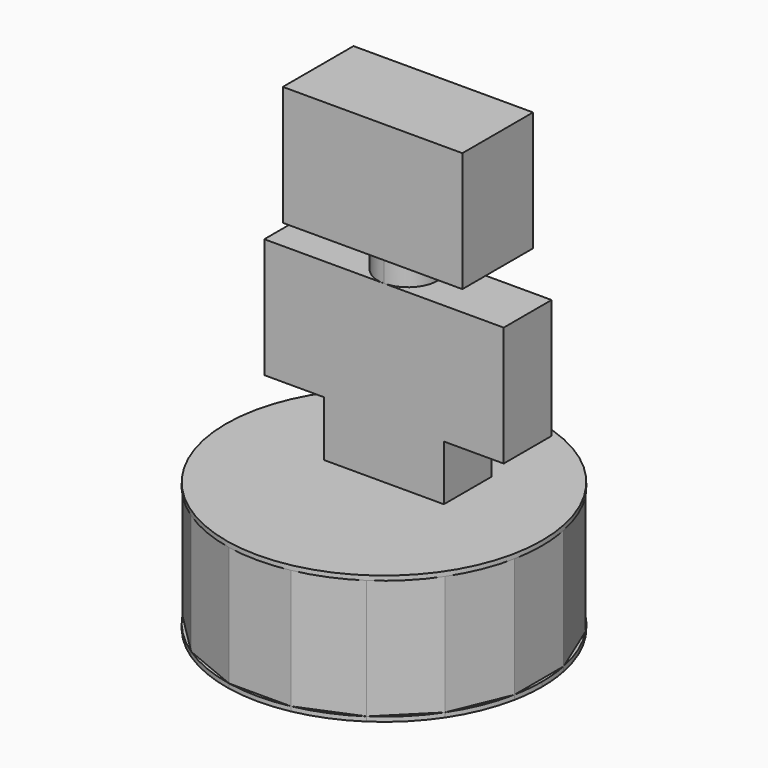
from build123d import *

# Parameters (mm, degrees)
F3_W      = 125
F3_H      = 62.5
F4_DEPTH  = 4.7625
F5_DEPTH  = 125
F6_R      = 165.0380183748
F7_DEPTH  = 4.7625
F8_DEPTH  = 386
F11_DEPTH = 62.5
F13_DEPTH = 31.25
F14_W     = 187.5
F14_H     = 92.25
F15_DEPTH = 125


# Not quite as in the source:
# - a length typed as a fraction of an inch, garbled in the dataset ("3 / 203.2 mm" for 3/8 in), is restored
# - a feature names something its author has since deleted; it is built from what else it names


with BuildPart() as f4:
    # F3 (on Top) → F4 (new body)
    with BuildSketch(Plane.XY):
        with BuildLine():
            ThreePointArc((161.8668591289, -32.1973201496), (164.2433152069, -16.1765546068), (165.0380183748, 0))
            ThreePointArc((165.0380183748, 0), (164.2433152069, 16.1765546068), (161.8668591289, 32.1973201496))
            Line((161.8668591289, 32.1973201496), (161.8668591289, -32.1973201496))
        make_face()
        with BuildLine():
            Line((137.2240971533, 91.6902103256), (161.8668591289, 32.1973201496))
            ThreePointArc((161.8668591289, 32.1973201496), (152.4752472627, 63.1573153424), (137.2240971533, 91.6902103256))
        make_face()
        Polygon((161.8668591289, -32.1973201496), (161.8668591289, 32.1973201496), (137.2240971533, 91.6902103256), (91.6902103256, 137.2240971533), (32.1973201496, 161.8668591289), (-32.1973201496, 161.8668591289), (-91.6902103256, 137.2240971533), (-137.2240971533, 91.6902103256), (-161.8668591289, 32.1973201496), (-161.8668591289, -32.1973201496), (-137.2240971533, -91.6902103256), (-91.6902103256, -137.2240971533), (-32.1973201496, -161.8668591289), (32.1973201496, -161.8668591289), (91.6902103256, -137.2240971533), (137.2240971533, -91.6902103256), align=None)
        with Locations((0, 31.25)):
            Rectangle(F3_W, F3_H, mode=Mode.SUBTRACT)
        with BuildLine():
            ThreePointArc((137.2240971533, -91.6902103256), (152.4752472627, -63.1573153424), (161.8668591289, -32.1973201496))
            Line((161.8668591289, -32.1973201496), (137.2240971533, -91.6902103256))
        make_face()
        with BuildLine():
            Line((91.6902103256, 137.2240971533), (137.2240971533, 91.6902103256))
            ThreePointArc((137.2240971533, 91.6902103256), (116.6995019464, 116.6995019464), (91.6902103256, 137.2240971533))
        make_face()
        with BuildLine():
            ThreePointArc((91.6902103256, -137.2240971533), (116.6995019464, -116.6995019464), (137.2240971533, -91.6902103256))
            Line((137.2240971533, -91.6902103256), (91.6902103256, -137.2240971533))
        make_face()
        with BuildLine():
            Line((32.1973201496, 161.8668591289), (91.6902103256, 137.2240971533))
            ThreePointArc((91.6902103256, 137.2240971533), (63.1573153424, 152.4752472627), (32.1973201496, 161.8668591289))
        make_face()
        with BuildLine():
            ThreePointArc((32.1973201496, -161.8668591289), (63.1573153424, -152.4752472627), (91.6902103256, -137.2240971533))
            Line((91.6902103256, -137.2240971533), (32.1973201496, -161.8668591289))
        make_face()
        with BuildLine():
            Line((-32.1973201496, 161.8668591289), (32.1973201496, 161.8668591289))
            ThreePointArc((32.1973201496, 161.8668591289), (0, 165.0380183748), (-32.1973201496, 161.8668591289))
        make_face()
        with BuildLine():
            ThreePointArc((-32.1973201496, -161.8668591289), (0, -165.0380183748), (32.1973201496, -161.8668591289))
            Line((32.1973201496, -161.8668591289), (-32.1973201496, -161.8668591289))
        make_face()
        with BuildLine():
            Line((-91.6902103256, 137.2240971533), (-32.1973201496, 161.8668591289))
            ThreePointArc((-32.1973201496, 161.8668591289), (-63.1573153424, 152.4752472627), (-91.6902103256, 137.2240971533))
        make_face()
        with BuildLine():
            ThreePointArc((-91.6902103256, -137.2240971533), (-63.1573153424, -152.4752472627), (-32.1973201496, -161.8668591289))
            Line((-32.1973201496, -161.8668591289), (-91.6902103256, -137.2240971533))
        make_face()
        with BuildLine():
            Line((-137.2240971533, 91.6902103256), (-91.6902103256, 137.2240971533))
            ThreePointArc((-91.6902103256, 137.2240971533), (-116.6995019464, 116.6995019464), (-137.2240971533, 91.6902103256))
        make_face()
        with BuildLine():
            ThreePointArc((-137.2240971533, -91.6902103256), (-116.6995019464, -116.6995019464), (-91.6902103256, -137.2240971533))
            Line((-91.6902103256, -137.2240971533), (-137.2240971533, -91.6902103256))
        make_face()
        with BuildLine():
            Line((-161.8668591289, 32.1973201496), (-137.2240971533, 91.6902103256))
            ThreePointArc((-137.2240971533, 91.6902103256), (-152.4752472627, 63.1573153424), (-161.8668591289, 32.1973201496))
        make_face()
        with BuildLine():
            ThreePointArc((-161.8668591289, -32.1973201496), (-152.4752472627, -63.1573153424), (-137.2240971533, -91.6902103256))
            Line((-137.2240971533, -91.6902103256), (-161.8668591289, -32.1973201496))
        make_face()
        with BuildLine():
            Line((-161.8668591289, -32.1973201496), (-161.8668591289, 32.1973201496))
            ThreePointArc((-161.8668591289, 32.1973201496), (-165.0380183748, 0), (-161.8668591289, -32.1973201496))
        make_face()
        with Locations((0, 31.25)):
            Rectangle(F3_W, F3_H)
    extrude(amount=-F4_DEPTH)

    # F3 (on Top) → F5 (join)
    with BuildSketch(Plane.XY):
        Polygon((161.8668591289, -32.1973201496), (161.8668591289, 32.1973201496), (137.2240971533, 91.6902103256), (91.6902103256, 137.2240971533), (32.1973201496, 161.8668591289), (-32.1973201496, 161.8668591289), (-91.6902103256, 137.2240971533), (-137.2240971533, 91.6902103256), (-161.8668591289, 32.1973201496), (-161.8668591289, -32.1973201496), (-137.2240971533, -91.6902103256), (-91.6902103256, -137.2240971533), (-32.1973201496, -161.8668591289), (32.1973201496, -161.8668591289), (91.6902103256, -137.2240971533), (137.2240971533, -91.6902103256), align=None)
        with Locations((0, 31.25)):
            Rectangle(F3_W, F3_H, mode=Mode.SUBTRACT)
        with Locations((0, 31.25)):
            Rectangle(F3_W, F3_H)
    extrude(amount=F5_DEPTH)

    # F6 (on face) → F7 (join)
    with BuildSketch(Plane.XY.offset(125)):
        Circle(F6_R)
    extrude(amount=F7_DEPTH)


with BuildPart() as f8:
    # F3 (on Top) → F8 (new body)
    with BuildSketch(Plane.XY):
        with Locations((0, 31.25)):
            Rectangle(F3_W, F3_H)
    extrude(amount=F8_DEPTH)


with BuildPart() as f4_1:
    add(f4.part)

    # F9: cut F8
    add(f8.part, mode=Mode.SUBTRACT)


with BuildPart() as f11:
    # F10 (on face) → F11 (new body)
    with BuildSketch(Plane.XZ.offset(-62.5)):
        Polygon((-62.5, 187.5), (-62.5, 0), (62.5, 0), (62.5, 187.5), (125, 187.5), (125, 312.5), (-125, 312.5), (-125, 187.5), align=None)
    extrude(amount=F11_DEPTH)


with BuildPart() as f13:
    # F12 (on face) → F13 (new body)
    with BuildSketch(Plane.XY.offset(312.5)):
        with BuildLine():
            ThreePointArc((9.8e-09, 0), (22.0970869155, 9.1529130914), (31.25, 31.25))
            ThreePointArc((31.25, 31.25), (22.0970869306, 53.3470868935), (5.24e-08, 62.5))
            ThreePointArc((5.24e-08, 62.5), (-31.25, 31.2500000213), (9.8e-09, 0))
        make_face()
    extrude(amount=F13_DEPTH)


with BuildPart() as f15:
    # F14 (on face) → F15 (new body)
    with BuildSketch(Plane.XY.offset(343.75)):
        with Locations((0, 31.25)):
            Rectangle(F14_W, F14_H)
    extrude(amount=F15_DEPTH)


solid = Compound([f4_1.part, f11.part, f13.part, f15.part])
